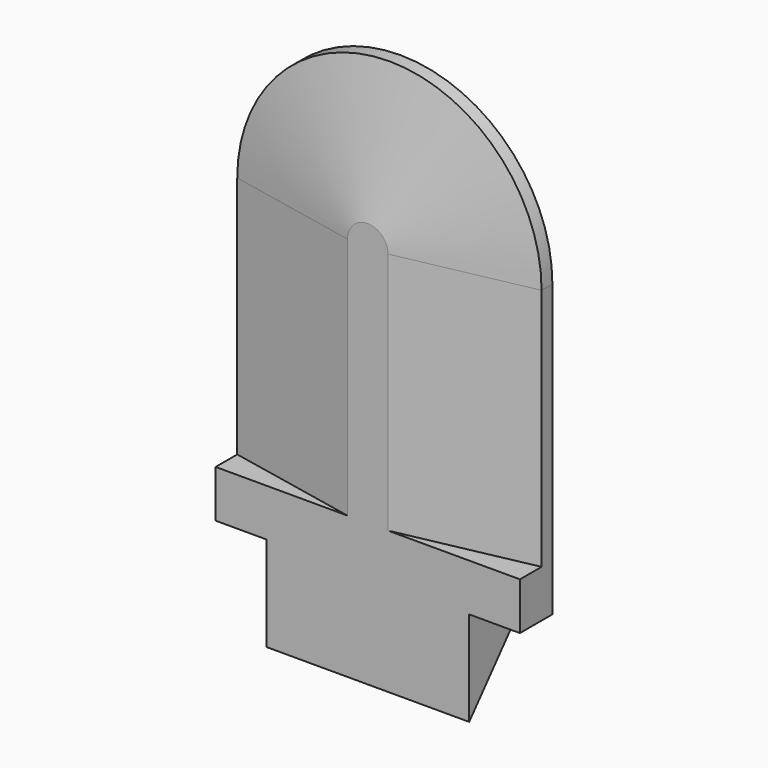
from build123d import *

# Parameters (mm, degrees)
F1_DEPTH = 6
F2_SIZE2 = 4
F2_SIZE  = 19.5
F3_W     = 45
F3_H     = 7
F4_DEPTH = 6
F5_W     = 30
F5_H     = 6
F6_DEPTH = 14
F7_W     = 30
F7_H     = 14
F8_DEPTH = 6
F9_SIZE2 = 11.99999
F9_SIZE  = 13.99999


# Not quite as in the source:
# - a fillet or chamfer is up to 0.001 mm smaller than in the source, because OpenCascade refuses the exact size


with BuildPart() as f1:
    # F0 (on Front) → F1 (new body)
    with BuildSketch(Plane.XZ):
        with BuildLine():
            ThreePointArc((0, 44), (-15.9099025767, 37.4099025767), (-22.5, 21.5))
            Line((-22.5, 21.5), (0, 21.5))
            Line((0, 21.5), (0, 44))
        make_face()
        with BuildLine():
            ThreePointArc((0, -1), (-15.9099025767, 5.5900974233), (-22.5, 21.5))
            Line((-22.5, 21.5), (-22.5, -21.5))
            Line((-22.5, -21.5), (0, -21.5))
            Line((0, -21.5), (0, -1))
        make_face()
        with BuildLine():
            Line((0, 21.5), (-22.5, 21.5))
            ThreePointArc((-22.5, 21.5), (-15.9099025767, 5.5900974233), (0, -1))
            Line((0, -1), (0, 21.5))
        make_face()
        with BuildLine():
            Line((0, 44), (0, 21.5))
            Line((0, 21.5), (22.5, 21.5))
            ThreePointArc((22.5, 21.5), (15.9099025767, 37.4099025767), (0, 44))
        make_face()
        with BuildLine():
            Line((22.5, 21.5), (0, 21.5))
            Line((0, 21.5), (0, -1))
            ThreePointArc((0, -1), (15.9099025767, 5.5900974233), (22.5, 21.5))
        make_face()
        with BuildLine():
            ThreePointArc((22.5, 21.5), (15.9099025767, 5.5900974233), (0, -1))
            Line((0, -1), (0, -21.5))
            Line((0, -21.5), (22.5, -21.5))
            Line((22.5, -21.5), (22.5, 21.5))
        make_face()
    extrude(amount=F1_DEPTH)

    # F2
    f2_edges = [f1.edges().sort_by_distance(p)[0] for p in [
        (0, -6, 44),
    ]]
    f2_side = f1.faces().sort_by_distance((0, -6, 9.043566))[0]
    chamfer(f2_edges, length=F2_SIZE, length2=F2_SIZE2, reference=f2_side)

    # F3 (on face) → F4 (join)
    with BuildSketch(Plane(origin=(0, 0, 0), x_dir=(-1, 0, 0), z_dir=(0, 1, 0))):
        with Locations((0, -18)):
            Rectangle(F3_W, F3_H)
    extrude(amount=-F4_DEPTH)

    # F5 (on face) → F6 (join)
    with BuildSketch(Plane(origin=(0, 0, -21.5), x_dir=(1, 0, 0), z_dir=(0, 0, -1))):
        with Locations((0, 3)):
            Rectangle(F5_W, F5_H)
    extrude(amount=F6_DEPTH)

    # F7 (on face) → F8 (join)
    with BuildSketch(Plane(origin=(0, 0, 0), x_dir=(-1, 0, 0), z_dir=(0, 1, 0))):
        with Locations((0, -28.5)):
            Rectangle(F7_W, F7_H)
    extrude(amount=F8_DEPTH)

    # F9 (size 14 and 12 in the source; OpenCascade refuses exactly that, so slightly less here)
    f9_edges = [f1.edges().sort_by_distance(p)[0] for p in [
        (0, 6, -35.5),
    ]]
    f9_side = f1.faces().sort_by_distance((0, 6, -28.5))[0]
    chamfer(f9_edges, length=F9_SIZE, length2=F9_SIZE2, reference=f9_side)


solid = f1.part
